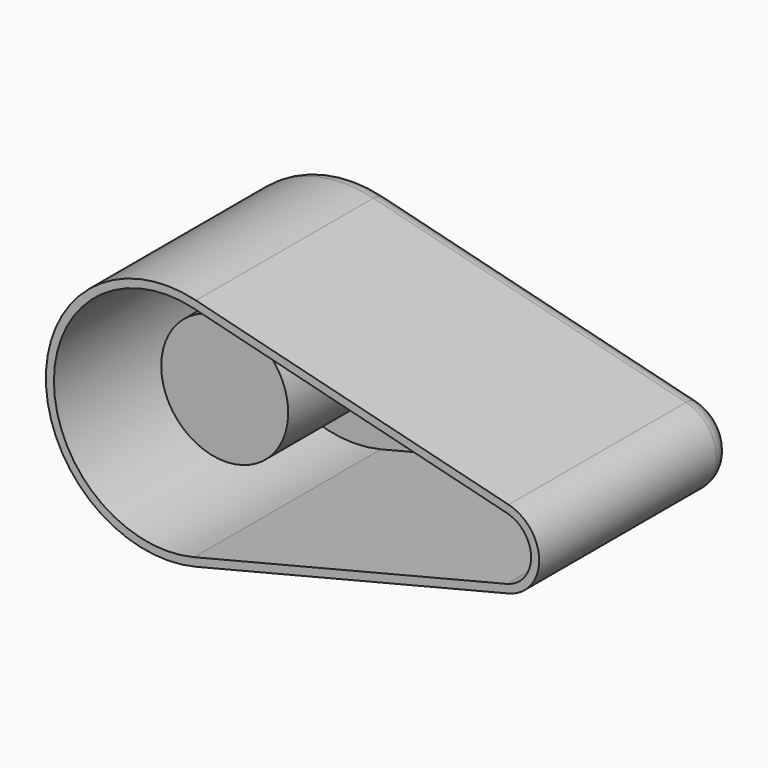
from build123d import *

# Parameters (mm, degrees)
F1_DEPTH     = 76.2
F2_R         = 17.4749230477
F2_R_2       = 8.76970131
F3_DEPTH     = 50.8
F4_T         = 2.54
F5_T5_DEPTH  = 101.6
F5_T7_DEPTH  = 101.6
F5_T14_ANGLE = 151.9275130641
F5_T16_ANGLE = 208.0724869359


# Not quite as in the source:
# - a fillet or chamfer that OpenCascade refuses, or shapes differently, is made with other operations: its cross-section is extruded or revolved along the edge and cut away or added
# - a shell that OpenCascade refuses in one call is made with other operations: the cavity is built on its own and cut out


with BuildPart() as f1:
    # F0 (on Front) → F1 (new body)
    with BuildSketch(Plane.XZ):
        with BuildLine():
            ThreePointArc((9.2406073139, -36.9624292555), (30.0306271884, -23.4472051782), (38.1, 0))
            ThreePointArc((38.1, 0), (30.0306271884, 23.4472051782), (9.2406073139, 36.9624292555))
            ThreePointArc((9.2406073139, 36.9624292555), (-38.1, 0), (9.2406073139, -36.9624292555))
        make_face()
        with BuildLine():
            ThreePointArc((9.2406073139, 36.9624292555), (30.0306271884, 23.4472051782), (38.1, 0))
            ThreePointArc((38.1, 0), (30.0306271884, -23.4472051782), (9.2406073139, -36.9624292555))
            Line((9.2406073139, -36.9624292555), (107.8070853287, -12.3208097518))
            ThreePointArc((107.8070853287, -12.3208097518), (92.0268828907, 0), (107.8070853287, 12.3208097518))
            Line((107.8070853287, 12.3208097518), (9.2406073139, 36.9624292555))
        make_face()
        with BuildLine():
            ThreePointArc((117.4268828907, 0), (114.7370919535, 7.8157350594), (107.8070853287, 12.3208097518))
            ThreePointArc((107.8070853287, 12.3208097518), (92.0268828907, 0), (107.8070853287, -12.3208097518))
            ThreePointArc((107.8070853287, -12.3208097518), (114.7370919535, -7.8157350594), (117.4268828907, 0))
        make_face()
    extrude(amount=F1_DEPTH)

    # F2 (on face) → F3 (cut)
    with BuildSketch(Plane(origin=(0, 0, 0), x_dir=(-1, 0, 0), z_dir=(0, 1, 0))):
        Circle(F2_R)
        with Locations((-104.7268828907, 0)):
            Circle(F2_R_2)
    extrude(amount=-F3_DEPTH, mode=Mode.SUBTRACT)

    # F4: shell of thickness 2.54, made by hand


with BuildPart() as f4_core1:
    # F4_t2: copy of F1
    add(f1.part)

    # the walls: a layer under each face that stays
    f4_faces = [f4_core1.faces().sort_by_distance(p)[0] for p in [
        (-38.1, -38.1, 0),
        (58.5238463213, -38.1, 24.6416195037),
        (58.5238463213, -38.1, -24.6416195037),
        (39.6634414453, 0, 0),
        (117.4268828907, -38.1, 0),
        (113.4965842007, -25.4, 0),
        (17.4749230477, -25.4, 0),
        (104.7268828907, -50.8, 0),
        (0, -50.8, 0),
    ]]
    thicken(f4_faces, amount=-F4_T, mode=Mode.SUBTRACT)

    # F4_s3 → F4_t4 (revolve, cut)
    with BuildSketch(Plane.XY):
        Polygon((95.9825815807, -50.7746), (93.4171815807, -50.8), (93.4171815807, -53.34), (95.9571815807, -53.34), align=None)
    revolve(axis=Axis((104.7268828907, -50.8, 0), (0, 1, 0)), mode=Mode.SUBTRACT)

    # F4_s5 → F4_t6 (revolve, cut)
    with BuildSketch(Plane.XY):
        Polygon((-17.4495230477, -50.7746), (-20.0149230477, -50.8), (-20.0149230477, -53.34), (-17.4749230477, -53.34), align=None)
    revolve(axis=Axis((0, -50.8, 0), (0, 1, 0)), mode=Mode.SUBTRACT)


with BuildPart() as f1_1:
    add(f1.part)

    # what is left inside the walls is the cavity
    f4_cavity = [f4_core1.part.solids().sort_by_distance(p)[0] for p in [
        (-35.5346, -51.646667, 0),
    ]]
    add(f4_cavity, mode=Mode.SUBTRACT)

    # F5: fillet of radius 6.35 on 5 edges, made by hand

    # F5_s1 → F5_t2 (revolve)
    with BuildSketch(Plane.XY):
        with BuildLine():
            ThreePointArc((95.9571815807, -44.45), (97.8170535202, -48.9401280605), (102.3071815807, -50.8))
            Line((102.3071815807, -50.8), (95.9571815807, -50.8))
            Line((95.9571815807, -50.8), (95.9571815807, -44.45))
        make_face()
    revolve(axis=Axis((104.7268828907, -50.8, 0), (0, 1, 0)))

    # F5_s3 → F5_t4 (revolve)
    with BuildSketch(Plane.XY):
        with BuildLine():
            ThreePointArc((-17.4749230477, -44.45), (-15.6150511082, -48.9401280605), (-11.1249230477, -50.8))
            Line((-11.1249230477, -50.8), (-17.4749230477, -50.8))
            Line((-17.4749230477, -50.8), (-17.4749230477, -44.45))
        make_face()
    revolve(axis=Axis((0, -50.8, 0), (0, 1, 0)))

    # F5_s6 → F5_t5 (cut)
    with BuildSketch(Plane(origin=(98.5664780148, 0, -24.6416195037), x_dir=(0, 1, 0), z_dir=(-0.9701425001, 0, 0.242535625))):
        with BuildLine():
            ThreePointArc((-6.35, -38.1), (-1.8598719395, -36.2401280605), (0, -31.75))
            Line((0, -31.75), (0, -38.1))
            Line((0, -38.1), (-6.35, -38.1))
        make_face()
    extrude(amount=F5_T5_DEPTH, mode=Mode.SUBTRACT)

    # F5_s8 → F5_t7 (cut)
    with BuildSketch(Plane(origin=(0, 0, 0), x_dir=(0, 1, 0), z_dir=(0.9701425001, 0, 0.242535625))):
        with BuildLine():
            ThreePointArc((-6.35, -38.1), (-1.8598719395, -36.2401280605), (0, -31.75))
            Line((0, -31.75), (0, -38.1))
            Line((0, -38.1), (-6.35, -38.1))
        make_face()
    extrude(amount=F5_T7_DEPTH, mode=Mode.SUBTRACT)

    # F5_s9 → F5_t10 (revolve, cut)
    with BuildSketch(Plane.XY):
        with BuildLine():
            ThreePointArc((89.6071815807, 0), (94.0973096412, -1.8598719395), (95.9571815807, -6.35))
            Line((95.9571815807, -6.35), (95.9571815807, 0))
            Line((95.9571815807, 0), (89.6071815807, 0))
        make_face()
    revolve(axis=Axis((104.7268828907, 0, 0), (0, 1, 0)), mode=Mode.SUBTRACT)

    # F5_s11 → F5_t12 (revolve, cut)
    with BuildSketch(Plane.XY):
        with BuildLine():
            ThreePointArc((-23.8249230477, 0), (-19.3347949872, -1.8598719395), (-17.4749230477, -6.35))
            Line((-17.4749230477, -6.35), (-17.4749230477, 0))
            Line((-17.4749230477, 0), (-23.8249230477, 0))
        make_face()
    revolve(axis=Axis((0, 0, 0), (0, 1, 0)), mode=Mode.SUBTRACT)

    # F5_s13 → F5_t14 (revolve, cut)
    with BuildSketch(Plane(origin=(98.5664780148, 0, 24.6416195037), x_dir=(0, 1, 0), z_dir=(-0.9701425001, 0, -0.242535625))):
        with BuildLine():
            ThreePointArc((0, 31.75), (-1.8598719395, 36.2401280605), (-6.35, 38.1))
            Line((-6.35, 38.1), (0, 38.1))
            Line((0, 38.1), (0, 31.75))
        make_face()
    revolve(axis=Axis((104.7268828907, 0, 0), (0, -1, 0)), revolution_arc=F5_T14_ANGLE, mode=Mode.SUBTRACT)

    # F5_s15 → F5_t16 (revolve, cut)
    with BuildSketch(Plane(origin=(0, 0, 0), x_dir=(0, 1, 0), z_dir=(0.9701425001, 0, -0.242535625))):
        with BuildLine():
            ThreePointArc((-6.35, 38.1), (-1.8598719395, 36.2401280605), (0, 31.75))
            Line((0, 31.75), (0, 38.1))
            Line((0, 38.1), (-6.35, 38.1))
        make_face()
    revolve(axis=Axis((0, 0, 0), (0, -1, 0)), revolution_arc=F5_T16_ANGLE, mode=Mode.SUBTRACT)


solid = f1_1.part
